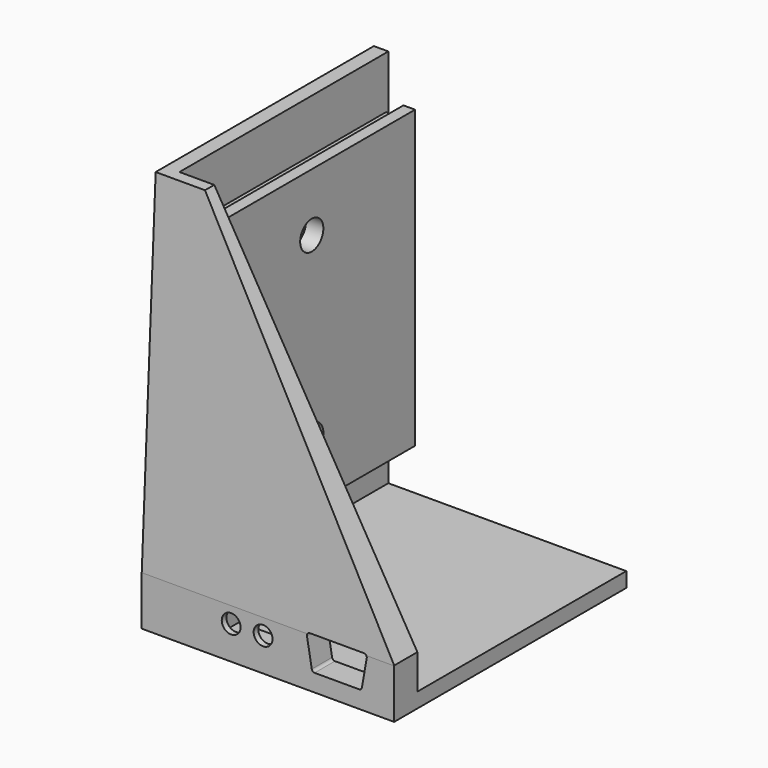
from build123d import *

# Parameters (mm, degrees)
F1_DEPTH  = 90
F3_DEPTH  = 10
F5_DEPTH  = 90
F6_SIZE   = 1
F8_DEPTH  = 8
F9_R      = 3.25
F10_DEPTH = 25
F12_DEPTH = 25
F11_W     = 31.5
F11_H     = 13.2
F13_DEPTH = 1.25
F14_R     = 5
F14_R_2   = 3
F15_DEPTH = 6
F16_DEPTH = 25


with BuildPart() as f1:
    # F0 (on Front) → F1 (new body)
    with BuildSketch(Plane.XZ):
        Polygon((5, 131), (0, 131), (0, 0), (5, 0), (5, 19), (11, 19), (11, 15), (15, 15), (15, 117), (11, 117), (11, 113), (5, 113), align=None)
        Polygon((5, 0), (0, 0), (0, -5.121096503), (87, -5.121096503), (87, 0), align=None)
    extrude(amount=F1_DEPTH)

    # F2 (on face) → F3 (join)
    with BuildSketch(Plane.XZ.offset(90)):
        Polygon((87, -5.121096503), (87, 0), (5, 0), (5, 19), (11, 19), (11, 15), (15, 15), (15, 117), (11, 117), (11, 113), (5, 113), (5, 131), (0, 131), (0, -5.121096503), align=None)
        Polygon((5, 0), (87, 0), (87, 12), (17, 131), (5, 131), (5, 113), (11, 113), (11, 117), (15, 117), (15, 15), (11, 15), (11, 19), (5, 19), align=None)
    extrude(amount=F3_DEPTH)

    # F4 (on face) → F5 (cut)
    with BuildSketch(Plane(origin=(0, 0, 0), x_dir=(0, -1, 0), z_dir=(-1, 0, 0))):
        Polygon((100, 131), (94, 131), (100, 11.878903497), align=None)
    extrude(amount=-F5_DEPTH, mode=Mode.SUBTRACT)

    # F6
    f6_edges = [f1.edges().sort_by_distance(p)[0] for p in [
        (8, 0, 113),
        (11, 0, 115),
        (13, 0, 117),
        (15, 0, 66),
        (13, 0, 15),
        (11, 0, 17),
        (8, 0, 19),
    ]]
    chamfer(f6_edges, length=F6_SIZE)

    # F7 (on face) → F8 (cut)
    with BuildSketch(Plane(origin=(0, -90, 0), x_dir=(-1, 0, 0), z_dir=(0, 1, 0))):
        Polygon((-25.625, 1.125), (-25.625, 11.625), (-44.025, 11.625), (-47.025, 9.075), (-47.025, 3.675), (-44.025, 1.125), align=None)
    extrude(amount=-F8_DEPTH, mode=Mode.SUBTRACT)

    # F9 (on face) → F10 (cut)
    with BuildSketch(Plane(origin=(0, -98, 0), x_dir=(-1, 0, 0), z_dir=(0, 1, 0))):
        with Locations((-41.825, 6.375)):
            Circle(F9_R)
        with Locations((-30.825, 6.375)):
            Circle(F9_R)
    extrude(amount=-F10_DEPTH, mode=Mode.SUBTRACT)

    # F11 (on face) → F12 (cut)
    with BuildSketch(Plane.XZ.offset(90)):
        with BuildLine():
            ThreePointArc((58.6058854217, 1.6786588252), (58.9474129273, 1.0847088218), (59.5910971765, 0.85))
            Line((59.5910971765, 0.85), (74.9089028235, 0.85))
            ThreePointArc((74.9089028235, 0.85), (75.5525870727, 1.0847088218), (75.8941145783, 1.6786588252))
            Line((75.8941145783, 1.6786588252), (77.5462884913, 11.1786588252))
            ThreePointArc((77.5462884913, 11.1786588252), (77.3263679147, 11.9936842492), (76.5610767365, 12.35))
            Line((76.5610767365, 12.35), (57.9389232635, 12.35))
            ThreePointArc((57.9389232635, 12.35), (57.1736320853, 11.9936842492), (56.9537115087, 11.1786588252))
            Line((56.9537115087, 11.1786588252), (58.6058854217, 1.6786588252))
        make_face()
    extrude(amount=F12_DEPTH, mode=Mode.SUBTRACT)

    # F11 (on face) → F13 (cut)
    with BuildSketch(Plane.XZ.offset(90)):
        with Locations((67.25, 6.6)):
            Rectangle(F11_W, F11_H)
        with BuildLine():
            Line((74.9089028235, 0.85), (59.5910971765, 0.85))
            ThreePointArc((59.5910971765, 0.85), (58.9474129273, 1.0847088218), (58.6058854217, 1.6786588252))
            Line((58.6058854217, 1.6786588252), (56.9537115087, 11.1786588252))
            ThreePointArc((56.9537115087, 11.1786588252), (57.1736320853, 11.9936842492), (57.9389232635, 12.35))
            Line((57.9389232635, 12.35), (76.5610767365, 12.35))
            ThreePointArc((76.5610767365, 12.35), (77.3263679147, 11.9936842492), (77.5462884913, 11.1786588252))
            Line((77.5462884913, 11.1786588252), (75.8941145783, 1.6786588252))
            ThreePointArc((75.8941145783, 1.6786588252), (75.5525870727, 1.0847088218), (74.9089028235, 0.85))
        make_face(mode=Mode.SUBTRACT)
    extrude(amount=F13_DEPTH, mode=Mode.SUBTRACT)

    # F14 (on face) → F15 (cut)
    with BuildSketch(Plane.YZ.offset(15)):
        with Locations((-45.5, 97)):
            Circle(F14_R)
        with Locations((-45.5, 97)):
            Circle(F14_R_2, mode=Mode.SUBTRACT)
        with Locations((-45.5, 35)):
            Circle(F14_R)
        with Locations((-45.5, 35)):
            Circle(F14_R_2, mode=Mode.SUBTRACT)
    extrude(amount=-F15_DEPTH, mode=Mode.SUBTRACT)

    # F16 (cut): faces of the model
    f16_faces = [f1.faces().sort_by_distance(p)[0] for p in [
        (15, -45.5, 97),
        (15, -45.5, 35),
    ]]
    extrude(f16_faces, amount=-F16_DEPTH, mode=Mode.SUBTRACT)


solid = f1.part
